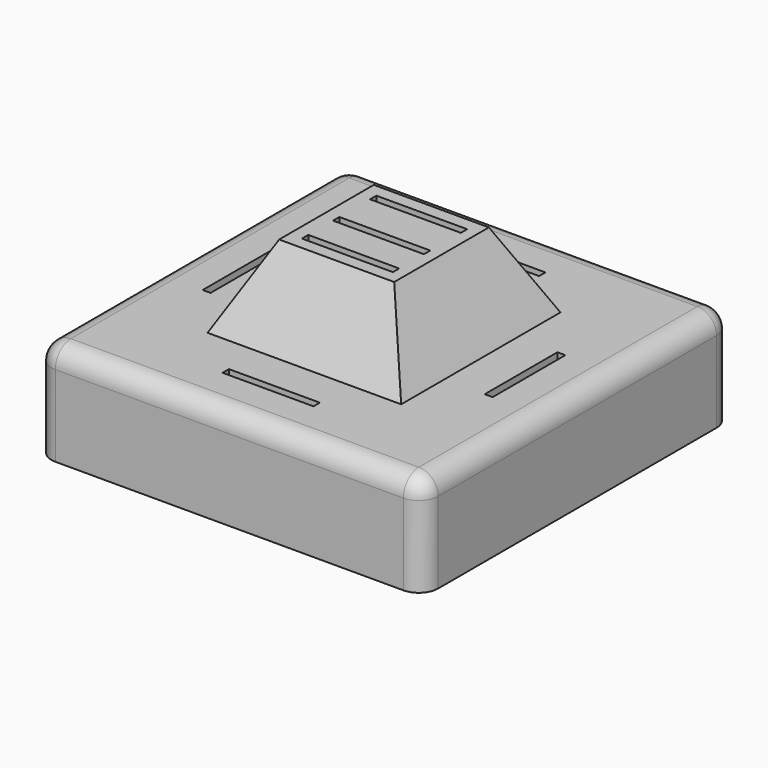
from build123d import *

# Parameters (mm, degrees)
F0_W         = 101.6
F0_H         = 101.6
F1_DEPTH     = 50.8
F2_W         = 50.8819408715
F2_H         = 52.3191291059
F6_R         = 5.08
F7_T1_DEPTH  = 58.42
F7_S5_W      = 5.08
F7_S5_H      = 5.08
F7_T6_DEPTH  = 5.08
F7_S11_W     = 5.08
F7_S11_H     = 5.08
F7_T12_DEPTH = 5.08
F7_S17_W     = 5.08
F7_S17_H     = 5.08
F7_T18_DEPTH = 5.08
F7_S23_W     = 5.08
F7_S23_H     = 5.08
F7_T24_DEPTH = 5.08
F8_W         = 36.9938705117
F8_H         = 32.6922610402
F9_DEPTH     = 43.434
F10_W        = 2.0828
F10_H        = 23.876
F10_W_2      = 23.876
F10_H_2      = 2.0828
F11_DEPTH    = 15.748
F12_W        = 11.7269940674
F12_H        = 2.0828
F12_W_2      = 12.1490059326
F13_DEPTH    = 15.748
F14_DEPTH    = 24.384


# Not quite as in the source:
# - a fillet or chamfer that OpenCascade refuses, or shapes differently, is made with other operations: its cross-section is extruded or revolved along the edge and cut away or added


with BuildPart() as f1:
    # F0 (on Top) → F1 (new body)
    with BuildSketch(Plane.XY):
        with Locations((3.134034574, 24.3160160567)):
            Rectangle(F0_W, F0_H)
    extrude(amount=F1_DEPTH)

    # F2 (on face) → F5 section 0
    with BuildSketch(Plane.XY.offset(50.8), mode=Mode.PRIVATE) as f5_s0:
        with Locations((3.134034574, 24.3160160567)):
            Rectangle(F2_W, F2_H)
    loft([Vertex(3.134034574, 24.3160160567, 101.6), f5_s0.sketch])

    # F6
    f6_edges = [f1.edges().sort_by_distance(p)[0] for p in [
        (3.134035, -26.483984, 50.8),
        (-47.665965, 24.316016, 50.8),
        (3.134035, 75.116016, 50.8),
        (53.934035, 24.316016, 50.8),
    ]]
    fillet(f6_edges, radius=F6_R)

    # F7: fillet of radius 5.08 on 4 edges, made by hand

    # F7_s2 → F7_t1 (cut)
    with BuildSketch(Plane.XY.offset(-12.7)):
        with BuildLine():
            ThreePointArc((-42.585965426, 75.1160160567), (-46.1780678744, 73.6281185051), (-47.665965426, 70.0360160567))
            Line((-47.665965426, 70.0360160567), (-47.665965426, 75.1160160567))
            Line((-47.665965426, 75.1160160567), (-42.585965426, 75.1160160567))
        make_face()
        with BuildLine():
            ThreePointArc((-47.665965426, -21.4039839433), (-46.1780678744, -24.9960863917), (-42.585965426, -26.4839839433))
            Line((-42.585965426, -26.4839839433), (-47.665965426, -26.4839839433))
            Line((-47.665965426, -26.4839839433), (-47.665965426, -21.4039839433))
        make_face()
        with BuildLine():
            ThreePointArc((53.934034574, -21.4039839433), (52.4461370225, -24.9960863917), (48.854034574, -26.4839839433))
            Line((48.854034574, -26.4839839433), (53.934034574, -26.4839839433))
            Line((53.934034574, -26.4839839433), (53.934034574, -21.4039839433))
        make_face()
        with BuildLine():
            ThreePointArc((48.854034574, 75.1160160567), (52.4461370225, 73.6281185051), (53.934034574, 70.0360160567))
            Line((53.934034574, 70.0360160567), (53.934034574, 75.1160160567))
            Line((53.934034574, 75.1160160567), (48.854034574, 75.1160160567))
        make_face()
    extrude(amount=F7_T1_DEPTH, mode=Mode.SUBTRACT)


with BuildPart() as f7_tool4:
    # F7_s5 → F7_t6 (new body)
    with BuildSketch(Plane.XZ.offset(-70.0360160567)):
        with Locations((51.394034574, 48.26)):
            Rectangle(F7_S5_W, F7_S5_H)
    extrude(amount=-F7_T6_DEPTH)

    # F7_s7 → F7_t8 (revolve, cut)
    with BuildSketch(Plane(origin=(48.854034574, 70.0360160567, 45.72), x_dir=(-0.7071067812, 0, -0.7071067812), z_dir=(0.7071067812, 0, -0.7071067812))):
        with BuildLine():
            ThreePointArc((0, -5.08), (5.08, 0), (0, 5.08))
            Line((0, 5.08), (0, -5.08))
        make_face()
    revolve(axis=Axis((48.854034574, 70.0360160567, 45.72), (0, 1, 0)), mode=Mode.SUBTRACT)


with BuildPart() as f1_1:
    add(f1.part)

    # F7_t3: cut F7_tool4
    add(f7_tool4.part, mode=Mode.SUBTRACT)


with BuildPart() as f7_tool10:
    # F7_s11 → F7_t12 (new body)
    with BuildSketch(Plane.YZ.offset(48.854034574)):
        with Locations((-23.9439839433, 48.26)):
            Rectangle(F7_S11_W, F7_S11_H)
    extrude(amount=F7_T12_DEPTH)

    # F7_s13 → F7_t14 (revolve, cut)
    with BuildSketch(Plane(origin=(48.854034574, -21.4039839433, 45.72), x_dir=(0, 0.7071067812, -0.7071067812), z_dir=(0, -0.7071067812, -0.7071067812))):
        with BuildLine():
            ThreePointArc((0, -5.08), (5.08, 0), (0, 5.08))
            Line((0, 5.08), (0, -5.08))
        make_face()
    revolve(axis=Axis((48.854034574, -21.4039839433, 45.72), (1, 0, 0)), mode=Mode.SUBTRACT)


with BuildPart() as f1_2:
    add(f1_1.part)

    # F7_t9: cut F7_tool10
    add(f7_tool10.part, mode=Mode.SUBTRACT)


with BuildPart() as f7_tool16:
    # F7_s17 → F7_t18 (new body)
    with BuildSketch(Plane.YZ.offset(-42.585965426)):
        with Locations((-23.9439839433, 48.26)):
            Rectangle(F7_S17_W, F7_S17_H)
    extrude(amount=-F7_T18_DEPTH)

    # F7_s19 → F7_t20 (revolve, cut)
    with BuildSketch(Plane(origin=(-42.585965426, -21.4039839433, 45.72), x_dir=(0, 0.7071067812, -0.7071067812), z_dir=(0, 0.7071067812, 0.7071067812))):
        with BuildLine():
            ThreePointArc((0, -5.08), (5.08, 0), (0, 5.08))
            Line((0, 5.08), (0, -5.08))
        make_face()
    revolve(axis=Axis((-42.585965426, -21.4039839433, 45.72), (-1, 0, 0)), mode=Mode.SUBTRACT)


with BuildPart() as f1_3:
    add(f1_2.part)

    # F7_t15: cut F7_tool16
    add(f7_tool16.part, mode=Mode.SUBTRACT)


with BuildPart() as f7_tool22:
    # F7_s23 → F7_t24 (new body)
    with BuildSketch(Plane.XZ.offset(-70.0360160567)):
        with Locations((-45.125965426, 48.26)):
            Rectangle(F7_S23_W, F7_S23_H)
    extrude(amount=-F7_T24_DEPTH)

    # F7_s25 → F7_t26 (revolve, cut)
    with BuildSketch(Plane(origin=(-42.585965426, 70.0360160567, 45.72), x_dir=(0.7071067812, 0, -0.7071067812), z_dir=(0.7071067812, 0, 0.7071067812))):
        with BuildLine():
            ThreePointArc((0, -5.08), (5.08, 0), (0, 5.08))
            Line((0, 5.08), (0, -5.08))
        make_face()
    revolve(axis=Axis((-42.585965426, 70.0360160567, 45.72), (0, 1, 0)), mode=Mode.SUBTRACT)


with BuildPart() as f1_4:
    add(f1_3.part)

    # F7_t21: cut F7_tool22
    add(f7_tool22.part, mode=Mode.SUBTRACT)

    # F8 (on Front) → F9 (cut)
    with BuildSketch(Plane.XZ):
        with Locations((2.3658862337, 87.7631418407)):
            Rectangle(F8_W, F8_H)
    extrude(amount=-F9_DEPTH, mode=Mode.SUBTRACT)

    # F10 (on face) → F11 (cut)
    with BuildSketch(Plane.XY.offset(50.8)):
        with Locations((-33.924565426, 24.3160160567)):
            Rectangle(F10_W, F10_H)
        with Locations((3.134034574, 61.3746160567)):
            Rectangle(F10_W_2, F10_H_2)
        with Locations((40.192634574, 24.3160160567)):
            Rectangle(F10_W, F10_H)
        with Locations((3.134034574, -12.7425839433)):
            Rectangle(F10_W_2, F10_H_2)
    extrude(amount=-F11_DEPTH, mode=Mode.SUBTRACT)

    # F12 (on face) → F13 (cut)
    with BuildSketch(Plane.XY.offset(71.4170113206)):
        with Locations((-2.7294624597, 35.4132379736)):
            Rectangle(F12_W, F12_H)
        with Locations((9.2085375403, 35.4132379736)):
            Rectangle(F12_W_2, F12_H)
        with Locations((9.2085375403, 13.0715451534)):
            Rectangle(F12_W_2, F12_H)
        with Locations((-2.7294624597, 13.0715451534)):
            Rectangle(F12_W, F12_H)
        with Locations((-2.7294624597, 23.2746160567)):
            Rectangle(F12_W, F12_H)
        with Locations((9.2085375403, 23.2746160567)):
            Rectangle(F12_W_2, F12_H)
    extrude(amount=-F13_DEPTH, mode=Mode.SUBTRACT)

    # F0 (on Top) → F14 (cut)
    with BuildSketch(Plane.XY):
        with Locations((3.134034574, 24.3160160567)):
            Rectangle(F0_W, F0_H)
    extrude(amount=F14_DEPTH, mode=Mode.SUBTRACT)


solid = f1_4.part
